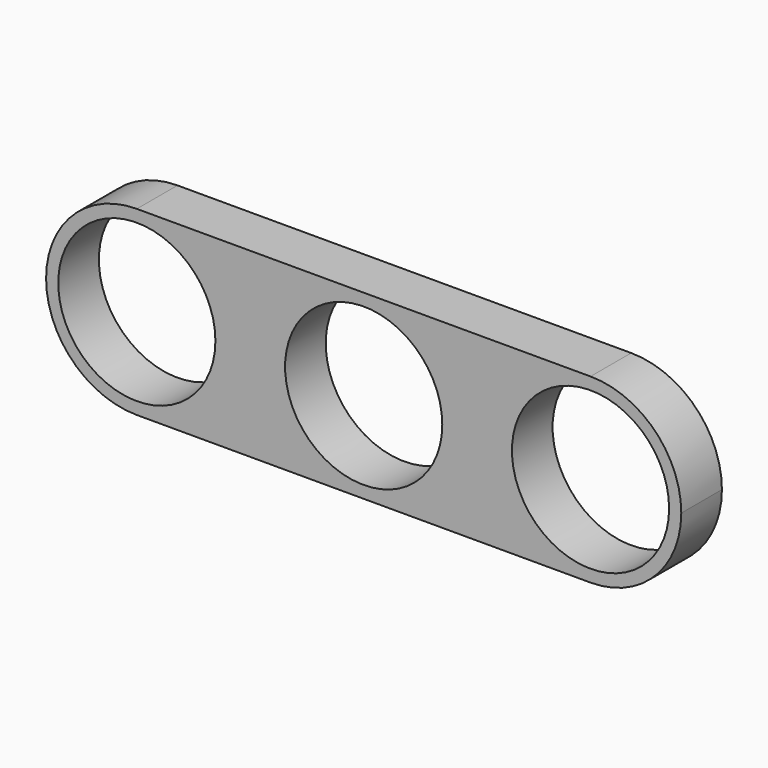
from build123d import *

# Parameters (mm, degrees)
F0_R     = 10.9982
F0_R_2   = 11
F1_DEPTH = 7.112


# Not quite as in the source:
# - a feature names something its author has since deleted; it is built from what else it names


with BuildPart() as f1:
    # F0 (on Front) → F1 (new body)
    with BuildSketch(Plane.XZ):
        with BuildLine():
            ThreePointArc((44.45, 0), (40.7302561211, 8.9802561211), (31.75, 12.7))
            ThreePointArc((31.75, 12.7), (19.05, 0), (31.75, -12.7))
            ThreePointArc((31.75, -12.7), (40.7302561211, -8.9802561211), (44.45, 0))
        make_face()
        with Locations((31.75, 0)):
            Circle(F0_R, mode=Mode.SUBTRACT)
        with BuildLine():
            ThreePointArc((-31.75, -12.7), (-22.7697438789, -8.9802561211), (-19.05, 0))
            ThreePointArc((-19.05, 0), (-22.7697438789, 8.9802561211), (-31.75, 12.7))
            ThreePointArc((-31.75, 12.7), (-44.45, 0), (-31.75, -12.7))
        make_face()
        with Locations((-31.75, 0)):
            Circle(F0_R, mode=Mode.SUBTRACT)
        with BuildLine():
            ThreePointArc((-31.75, 12.7), (-22.7697438789, 8.9802561211), (-19.05, 0))
            ThreePointArc((-19.05, 0), (-22.7697438789, -8.9802561211), (-31.75, -12.7))
            Line((-31.75, -12.7), (31.75, -12.7))
            ThreePointArc((31.75, -12.7), (19.05, 0), (31.75, 12.7))
            Line((31.75, 12.7), (-31.75, 12.7))
        make_face()
        Circle(F0_R_2, mode=Mode.SUBTRACT)
    extrude(amount=F1_DEPTH)


solid = f1.part
